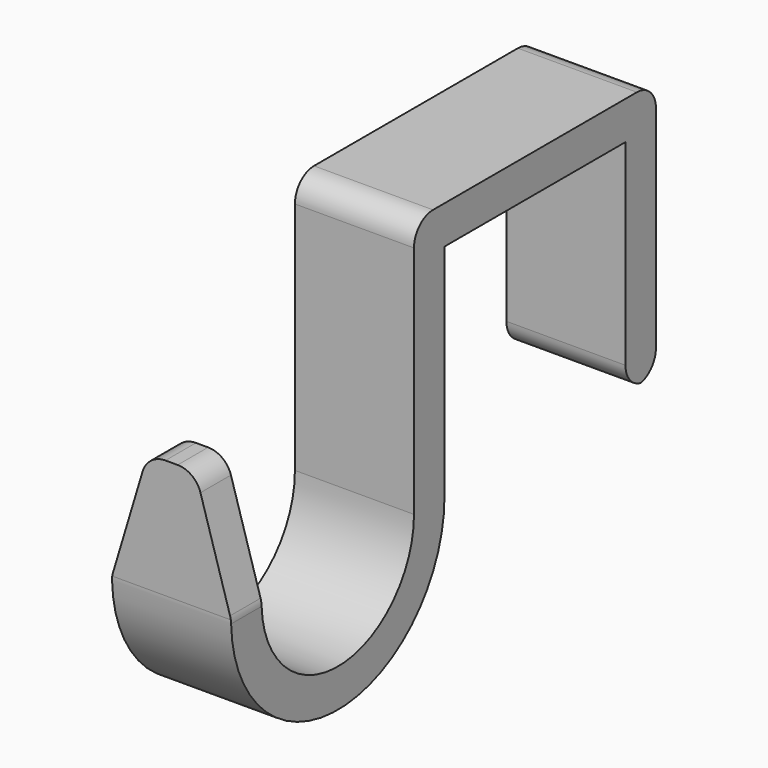
from build123d import *

# Parameters (mm, degrees)
F0_W        = 3.2
F0_H        = 10
F1_DEPTH    = 10
F2_SIZE2    = 10
F2_SIZE     = 3
F3_T1_DEPTH = 10.6403065089
F3_T3_DEPTH = 4.667688363
F3_T5_DEPTH = 20


# Not quite as in the source:
# - a fillet or chamfer that OpenCascade refuses, or shapes differently, is made with other operations: its cross-section is extruded or revolved along the edge and cut away or added


with BuildPart() as f1:
    # F0 (on Right) → F1 (new body)
    with BuildSketch(Plane.YZ):
        with Locations((-30.3, 5)):
            Rectangle(F0_W, F0_H)
        with BuildLine():
            Line((-9.5, 0), (-12.7, 0))
            ThreePointArc((-12.7, 0), (-20.7, -8), (-28.7, 0))
            Line((-28.7, 0), (-31.9, 0))
            ThreePointArc((-31.9, 0), (-20.7, -11.2), (-9.5, 0))
        make_face()
        Polygon((-12.7, 21.7), (-12.7, 0), (-9.5, 0), (-9.5, 18.5), (9.5, 18.5), (9.5, 0), (12.7, 0), (12.7, 21.7), align=None)
    extrude(amount=F1_DEPTH)

    # F2
    f2_edges = [f1.edges().sort_by_distance(p)[0] for p in [
        (10, -30.3, 10),
        (0, -30.3, 10),
    ]]
    f2_side = f1.faces().sort_by_distance((5, -30.3, 10))[0]
    chamfer(f2_edges, length=F2_SIZE, length2=F2_SIZE2, reference=f2_side)

    # F3: fillet of radius 2 on 8 edges, made by hand

    # F3_s2 → F3_t1 (cut)
    with BuildSketch(Plane.XZ.offset(24.9798467455)):
        with BuildLine():
            ThreePointArc((5.5119386982, 10), (6.7057997575, 9.6045858566), (7.4275912687, 8.5746957711))
            Line((7.4275912687, 8.5746957711), (7, 10))
            Line((7, 10), (5.5119386982, 10))
        make_face()
        with BuildLine():
            ThreePointArc((4.4880613018, 10), (3.2942002425, 9.6045858566), (2.5724087313, 8.5746957711))
            Line((2.5724087313, 8.5746957711), (3, 10))
            Line((3, 10), (4.4880613018, 10))
        make_face()
    extrude(amount=F3_T1_DEPTH, mode=Mode.SUBTRACT)

    # F3_s4 → F3_t3 (cut)
    with BuildSketch(Plane.XZ.offset(27.9661558185)):
        with BuildLine():
            ThreePointArc((9.9156525704, 0.2811580985), (9.978800791, -0.0031113832), (10, -0.2935376726))
            Line((10, -0.2935376726), (10, 0))
            Line((10, 0), (9.9156525704, 0.2811580985))
        make_face()
        with BuildLine():
            ThreePointArc((0.0843474296, 0.2811580985), (0.021199209, -0.0031113832), (0, -0.2935376726))
            Line((0, -0.2935376726), (0, 0))
            Line((0, 0), (0.0843474296, 0.2811580985))
        make_face()
    extrude(amount=F3_T3_DEPTH, mode=Mode.SUBTRACT)

    # F3_s6 → F3_t5 (cut)
    with BuildSketch(Plane.YZ.offset(-5)):
        with BuildLine():
            ThreePointArc((-12.7, 19.7), (-12.1142135624, 21.1142135624), (-10.7, 21.7))
            Line((-10.7, 21.7), (-12.7, 21.7))
            Line((-12.7, 21.7), (-12.7, 19.7))
        make_face()
        with BuildLine():
            ThreePointArc((10.7, 21.7), (12.1142135624, 21.1142135624), (12.7, 19.7))
            Line((12.7, 19.7), (12.7, 21.7))
            Line((12.7, 21.7), (10.7, 21.7))
        make_face()
        with BuildLine():
            ThreePointArc((9.5, 2), (10.0857864376, 0.5857864376), (11.5, 0))
            Line((11.5, 0), (9.5, 0))
            Line((9.5, 0), (9.5, 2))
        make_face()
        with BuildLine():
            ThreePointArc((12.7, 2), (12.1142135624, 0.5857864376), (10.7, 0))
            Line((10.7, 0), (12.7, 0))
            Line((12.7, 0), (12.7, 2))
        make_face()
    extrude(amount=F3_T5_DEPTH, mode=Mode.SUBTRACT)


solid = f1.part
